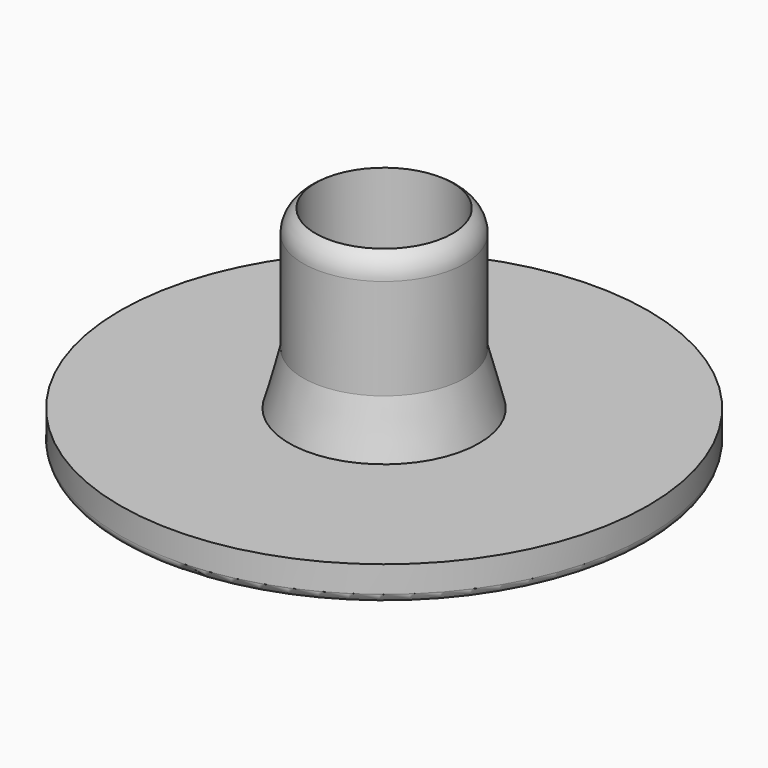
from build123d import *

# Parameters (mm, degrees)
F3_R     = 3.8930000325
F4_DEPTH = 12.001


# Not quite as in the source:
# - a fillet or chamfer that OpenCascade refuses, or shapes differently, is made with other operations: its cross-section is extruded or revolved along the edge and cut away or added


with BuildPart() as f1:
    # F0 (on Front) → F1 (revolve)
    with BuildSketch(Plane.XZ):
        with BuildLine():
            Line((0, 12), (0, 0))
            Line((0, 0), (14.5, 0))
            ThreePointArc((14.5, 0), (14.8535533906, 0.1464466094), (15, 0.5))
            Line((15, 0.5), (15, 2))
            Line((15, 2), (5.4, 2))
            Line((5.4, 2), (4.6, 5))
            Line((4.6, 5), (4.6, 12))
            Line((4.6, 12), (0, 12))
        make_face()
    revolve(axis=Axis((0, 0, 6), (0, 0, 1)))

    # F3 (on face) → F4 (cut, through all)
    with BuildSketch(Plane.XY.offset(12)):
        Circle(F3_R)
    extrude(amount=-F4_DEPTH, mode=Mode.SUBTRACT)

    # F5: fillet of radius 1.5 on 1 edges, made by hand

    # F5_s1 → F5_t2 (revolve, cut)
    with BuildSketch(Plane.XZ):
        with BuildLine():
            ThreePointArc((3.8930000325, 12), (4.4113923991, 11.4549383915), (4.6, 10.7267557389))
            Line((4.6, 10.7267557389), (4.6, 12))
            Line((4.6, 12), (3.8930000325, 12))
        make_face()
    revolve(axis=Axis((0, 0, 12), (0, 0, 1)), mode=Mode.SUBTRACT)


solid = f1.part
